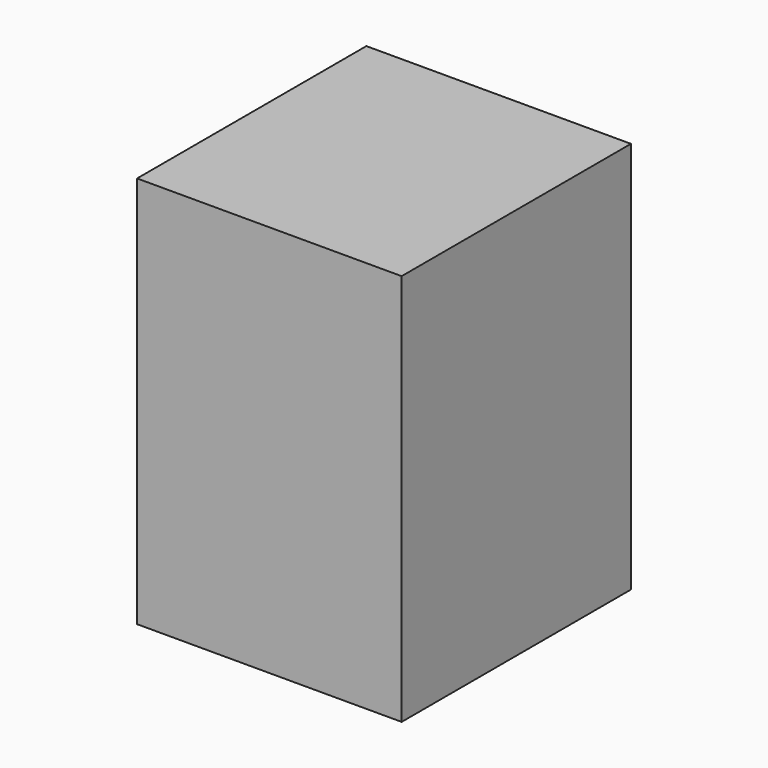
from build123d import *

# Parameters (mm, degrees)
F1_W     = 600
F1_H     = 650
F2_DEPTH = 890
F4_W     = 680
F4_H     = 970
F5_DEPTH = 3992


# Not quite as in the source:
# - an extrude ends at something that could not be found from the text; its depth is read off the source's solid


with BuildPart() as f2:
    # F1 (on Top) → F2 (new body)
    with BuildSketch(Plane.XY):
        with Locations((-1167.5, 590)):
            Rectangle(F1_W, F1_H)
    extrude(amount=F2_DEPTH)

    # F4 (on face) → F5 (cut, through all)
    with BuildSketch(Plane(origin=(1467.5, 0, 0), x_dir=(0, -1, 0), z_dir=(-1, 0, 0))):
        with Locations((-25, 1445)):
            Rectangle(F4_W, F4_H)
    extrude(amount=F5_DEPTH, mode=Mode.SUBTRACT)


solid = f2.part
